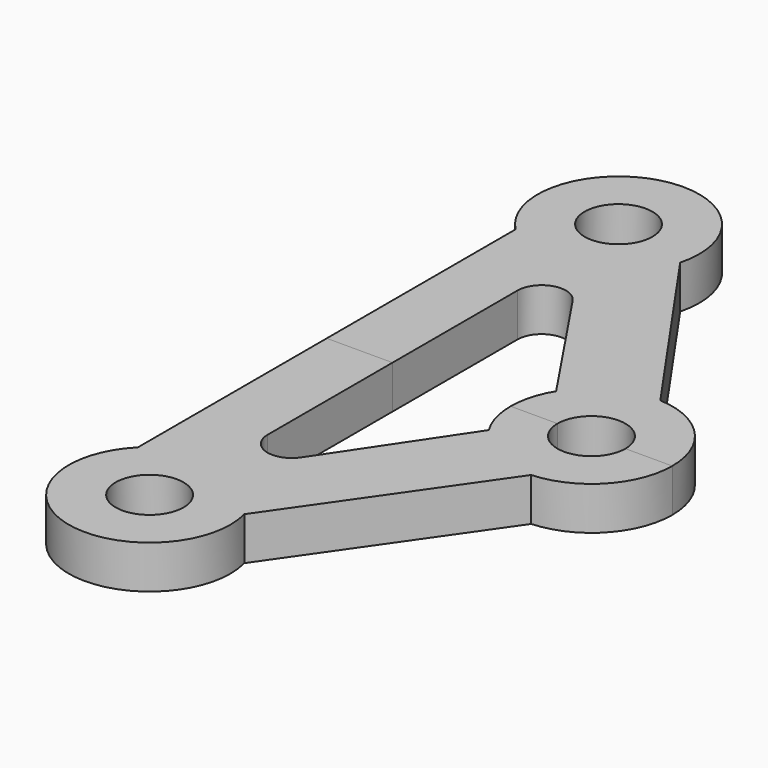
from build123d import *
from build123d import SkipClean  # not in build123d's __all__

# Parameters (mm, degrees)
F0_R     = 4
F1_DEPTH = 2.54


with BuildPart() as f1:
    # F0 (on Top) → F1 (new body, symmetric)
    with BuildSketch(Plane.XY):
        with BuildLine():
            Line((12.7523779158, 9.5117846914), (-2.9762470444, 32.0985170452))
            ThreePointArc((-2.9762470444, 32.0985170452), (-14.6529201579, 43.7315272534), (-18.9402122051, 27.8164165593))
            Line((-18.9402122051, 27.8164165593), (-18.9402122051, 0))
            Line((-18.9402122051, 0), (-11.187657958, 0))
            Line((-11.187657958, 0), (-11.187657958, 18.4020288289))
            ThreePointArc((-11.187657958, 18.4020288289), (-9.1615879854, 21.1358961189), (-5.9564906022, 19.9929435136))
            Line((-5.9564906022, 19.9929435136), (4.1191245614, 4.9599822668))
            ThreePointArc((4.1191245614, 4.9599822668), (3.0807470851, 2.5759836915), (2.725803411, 0))
            Line((2.725803411, 0), (8.250803411, 0))
            ThreePointArc((8.250803411, 0), (12.250803411, 4), (16.250803411, 0))
            Line((16.250803411, 0), (21.775803411, 0))
            ThreePointArc((21.775803411, 0), (19.1610538463, 6.5554606185), (12.7523779158, 9.5117846914))
        make_face()
        with Locations((-12.1852122247, 34.5317423344)):
            Circle(F0_R, mode=Mode.SUBTRACT)
    extrude(amount=F1_DEPTH, both=True)

    # F2: F1 across plane


with BuildPart() as f1_1:
    add(f1.part, clean=False)
    with SkipClean():  # cleaning this boolean's faces spoils the solid; the shape is the same uncleaned
        add(f1.part.mirror(Plane.XZ), clean=False)


solid = f1_1.part
